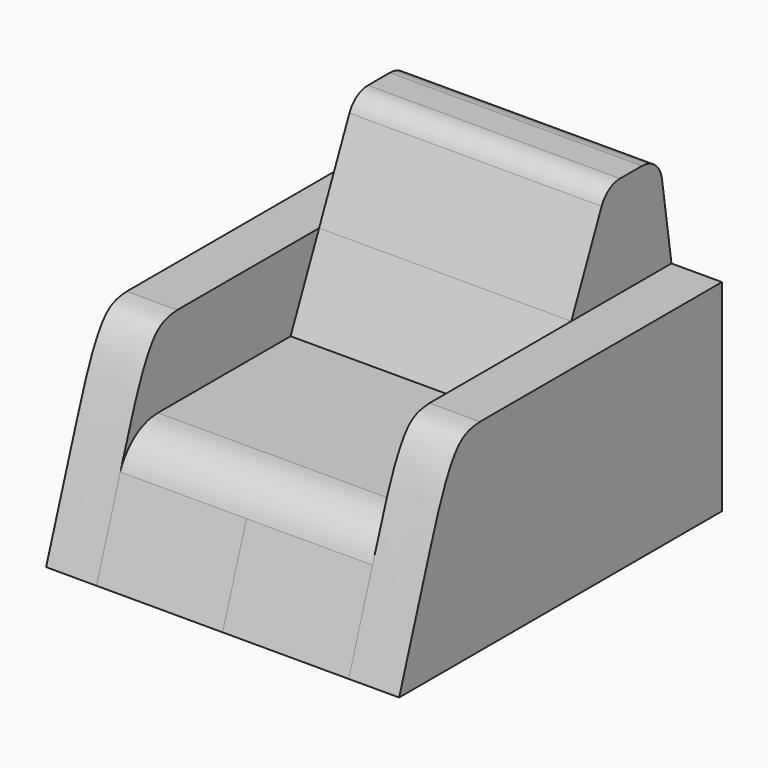
from build123d import *

# Parameters (mm, degrees)
F1_DEPTH    = 10
F3_DEPTH    = 25
F4_T1_DEPTH = 42.9731541067
F5_T1_DEPTH = 128.9574388021
F6_R        = 5


# Not quite as in the source:
# - a fillet or chamfer that OpenCascade refuses, or shapes differently, is made with other operations: its cross-section is extruded or revolved along the edge and cut away or added


with BuildPart() as f1:
    # F0 (on Right) → F1 (new body)
    with BuildSketch(Plane.YZ):
        with BuildLine():
            add(Edge.make_bspline(
                [(0, 0), (2.2442765195, 6.6212257172), (6.5959199803, 19.4597566844), (13.2513144203, 39.4417291966), (18.2658911198, 39.8565494945), (20, 40)],
                knots=[0, 0, 0, 0, 0.4106161004, 0.7961830249, 1, 1, 1, 1], degree=3))
            Line((0, 0), (80, 0))
            Line((80, 0), (80, 40))
            Line((80, 40), (20, 40))
        make_face()
    extrude(amount=F1_DEPTH)

    # F2 (on face) → F3 (join)
    with BuildSketch(Plane.YZ.offset(10)):
        with BuildLine():
            Line((0, 0), (80, 0))
            Line((80, 0), (80, 24))
            Line((80, 24), (80, 40))
            Line((80, 40), (55.1697723937, 40))
            Line((55.1697723937, 40), (48.1055903086, 24))
            Line((48.1055903086, 24), (8.1055903086, 24))
            add(Edge.make_bspline(
                [(6.8883897, 20.3932494068), (7.4606886756, 22.0855747763), (7.7861850662, 23.041763844), (8.1055903086, 24)],
                knots=[0.7039634953, 0.7039634953, 0.7039634953, 0.7039634953, 1, 1, 1, 1], degree=3))
            add(Edge.make_bspline(
                [(0, 0), (2.2153512314, 6.5358882555), (4.4307024628, 13.0717765111), (6.8883896999, 20.3932494068)],
                knots=[0, 0, 0, 0, 0.4053238875, 0.4053238875, 0.4053238875, 0.4053238875], degree=3))
        make_face()
        Polygon((55.1697723937, 40), (80, 40), (80, 60), (74, 60), (64, 60), align=None)
    extrude(amount=F3_DEPTH)

    # F4: fillet of radius 10 on 1 edges, made by hand

    # F4_s2 → F4_t1 (cut)
    with BuildSketch(Plane.YZ.offset(10)):
        with BuildLine():
            ThreePointArc((5.8068468985, 17.1881528422), (9.4498542284, 22.1207148199), (15.2866730275, 24.0004))
            Line((15.2866730275, 24.0004), (15.2866730275, 25.0006119097))
            ThreePointArc((15.2866730275, 25.0006119097), (11.696131668, 25.0002119097), (8.1055903086, 25.0002119097))
            Line((8.1055903086, 25.0002119097), (7.1567039525, 24.3162887089))
            ThreePointArc((7.1567039525, 24.3162887089), (6.0088321462, 20.9145484967), (4.8588642856, 17.5071400361))
            Line((4.8588642856, 17.5071400361), (5.8068468985, 17.1881528422))
        make_face()
    extrude(amount=F4_T1_DEPTH, mode=Mode.SUBTRACT)

    # F5: chamfer of 3 x 20 on 1 edges, made by hand

    # F5_s2 → F5_t1 (cut)
    with BuildSketch(Plane.YZ.offset(-41.9787194011)):
        Polygon((80, 40), (77, 60), (80, 60), align=None)
    extrude(amount=F5_T1_DEPTH, mode=Mode.SUBTRACT)

    # F6
    f6_edges = [f1.edges().sort_by_distance(p)[0] for p in [
        (22.5, 64, 60),
        (22.5, 77, 60),
    ]]
    fillet(f6_edges, radius=F6_R)

    # F7: F1 across face


with BuildPart() as f1_1:
    add(f1.part)
    add(f1.part.mirror(Plane(origin=(35, 49.9855810819, 20.3924452075), x_dir=(0, 1, 0), z_dir=(1, 0, 0))))


solid = f1_1.part
